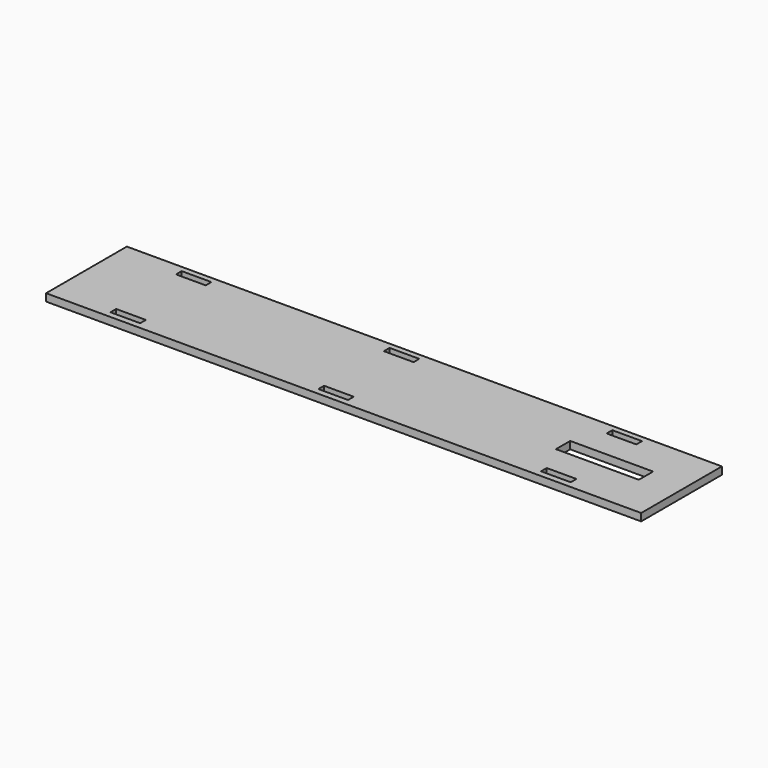
from build123d import *

# Parameters (mm, degrees)
F0_W     = 254.508
F0_H     = 43.18
F0_W_2   = 12.7
F0_H_2   = 3.048
F1_DEPTH = 3.175


# Not quite as in the source:
# - a feature names something its author has since deleted; it is built from what else it names


with BuildPart() as f1:
    # F0 (on Top) → F1 (new body)
    with BuildSketch(Plane.XY):
        with Locations((0.254, 0.1834339905)):
            Rectangle(F0_W, F0_H)
        with Locations((-95.25, -17.2155660095)):
            Rectangle(F0_W_2, F0_H_2, mode=Mode.SUBTRACT)
        with Locations((-6.35, -17.2155660095)):
            Rectangle(F0_W_2, F0_H_2, mode=Mode.SUBTRACT)
        with Locations((88.9, -17.2155660095)):
            Rectangle(F0_W_2, F0_H_2, mode=Mode.SUBTRACT)
        with Locations((-95.25, 17.8364339905)):
            Rectangle(F0_W_2, F0_H_2, mode=Mode.SUBTRACT)
        with Locations((-6.35, 17.8364339905)):
            Rectangle(F0_W_2, F0_H_2, mode=Mode.SUBTRACT)
        Polygon((78.9593234658, -3.1185660095), (76.4378011227, -3.1185660095), (76.4378011227, 4.5014339905), (78.9593234658, 4.5014339905), (111.8867844343, 4.5014339905), (111.8867844343, -3.1185660095), align=None, mode=Mode.SUBTRACT)
        with Locations((88.9, 17.8364339905)):
            Rectangle(F0_W_2, F0_H_2, mode=Mode.SUBTRACT)
    extrude(amount=F1_DEPTH)


solid = f1.part
